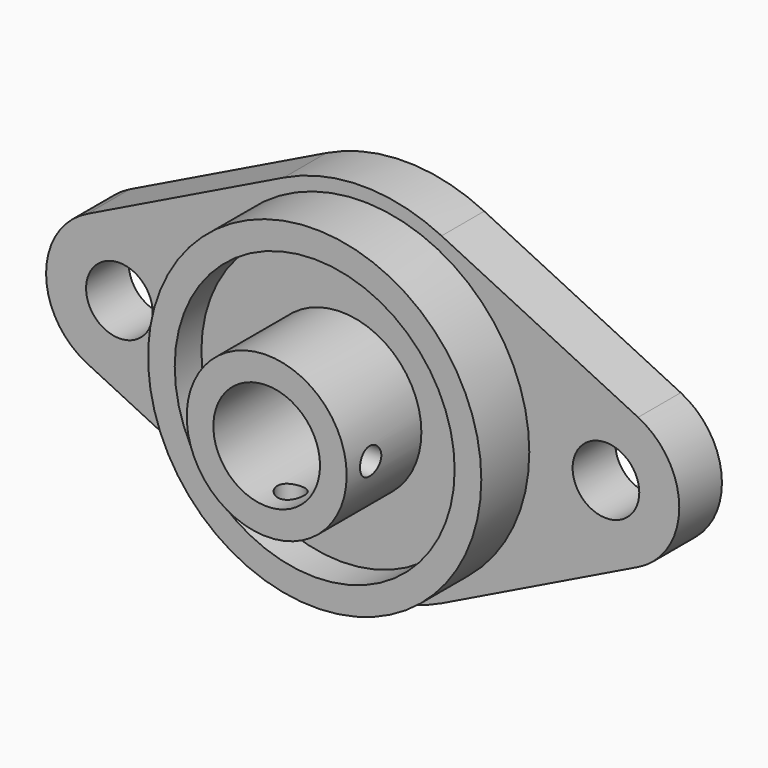
from build123d import *

# Parameters (mm, degrees)
F0_R     = 2.5
F1_DEPTH = 2
F2_R     = 12.5
F2_R_2   = 10.5
F3_DEPTH = 4.5
F4_R     = 6
F4_R_2   = 4
F5_DEPTH = 9
F6_DEPTH = 4.001
F7_DEPTH = 2
F8_R     = 1
F9_DEPTH = 13.501


# Not quite as in the source:
# - a pattern or mirror of a feature is missing from the dataset's text; its kind, count and spacing are read off the source's solid


with BuildPart() as f1:
    # F0 (on Front) → F1 (new body, symmetric)
    with BuildSketch(Plane.XZ):
        with BuildLine():
            Line((-5.9178082192, 12.133818273), (-20.6609589041, 4.9434074445))
            ThreePointArc((-20.6609589041, 4.9434074445), (-23.75, 0), (-20.6609589041, -4.9434074445))
            Line((-20.6609589041, -4.9434074445), (-5.9178082192, -12.133818273))
            ThreePointArc((-5.9178082192, -12.133818273), (0, -13.5), (5.9178082192, -12.133818273))
            Line((5.9178082192, -12.133818273), (20.6609589041, -4.9434074445))
            ThreePointArc((20.6609589041, -4.9434074445), (23.75, 0), (20.6609589041, 4.9434074445))
            Line((20.6609589041, 4.9434074445), (5.9178082192, 12.133818273))
            ThreePointArc((5.9178082192, 12.133818273), (0, 13.5), (-5.9178082192, 12.133818273))
        make_face()
        with Locations((-18.25, 0)):
            Circle(F0_R, mode=Mode.SUBTRACT)
        with Locations((18.25, 0)):
            Circle(F0_R, mode=Mode.SUBTRACT)
    extrude(amount=F1_DEPTH, both=True)

    # F2 (on face) → F3 (join)
    with BuildSketch(Plane.XZ.offset(2)):
        Circle(F2_R)
        Circle(F2_R_2, mode=Mode.SUBTRACT)
    extrude(amount=F3_DEPTH)

    # F4 (on face) → F5 (join)
    with BuildSketch(Plane.XZ.offset(2)):
        Circle(F4_R)
        Circle(F4_R_2, mode=Mode.SUBTRACT)
    extrude(amount=F5_DEPTH)

    # F4 (on face) → F6 (cut, through all)
    with BuildSketch(Plane.XZ.offset(2)):
        Circle(F4_R_2)
    extrude(amount=-F6_DEPTH, mode=Mode.SUBTRACT)


with BuildPart() as f7:
    # F7 (new): a face of the model
    f7_faces = [f1.part.faces().sort_by_distance(p)[0] for p in [
        (-10.2030151519, -2, 0),
    ]]
    extrude(f7_faces, amount=F7_DEPTH)


with BuildPart() as f1_1:
    add(f1.part)

    # F8 (on Top) → F9 (cut, through all)
    with BuildSketch(Plane.XY):
        with Locations((0, -8.75)):
            Circle(F8_R)
    f9 = extrude(amount=-F9_DEPTH, mode=Mode.SUBTRACT)

    # F9_copies: F9 across plane
    add(f9.mirror(Plane(origin=(0, 0, 0), x_dir=(-0.7071067098, 0, 0.7071068526), z_dir=(0.7071068526, 2.218e-07, 0.7071067098))), mode=Mode.SUBTRACT)


solid = Compound([f7.part, f1_1.part])
